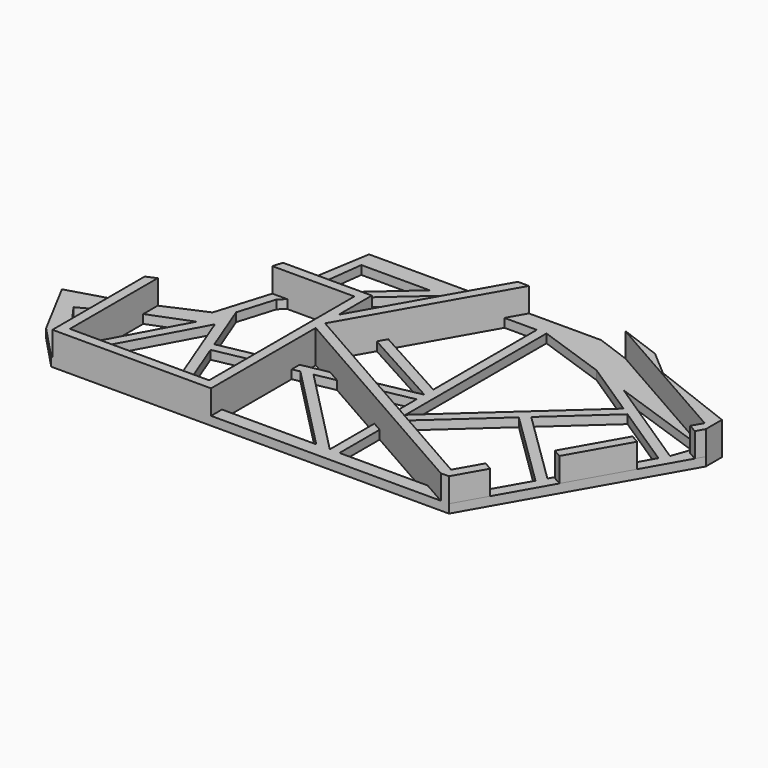
from build123d import *

# Parameters (mm, degrees)
F1_DEPTH      = 2.286
F4_DEPTH      = 2.287
F5_DEPTH      = 6.35
F5_DEPTH_BACK = 2.286


# Not quite as in the source:
# - a feature names something its author has since deleted; it is built from what else it names


with BuildPart() as f1:
    # F0 (on Top) → F1 (new body)
    with BuildSketch(Plane.XY):
        Polygon((-39.7502322496, -19.8751161248), (-31.0001806734, -29.1251689516), (73.3058652154, -29.1251689516), (101.3186621261, 20.063493978), (101.3186621261, 25.3395497125), (78.8771229202, 34.0285638846), (72.3271246897, 39.6729167182), (52.3297434038, 47.023841916), (50.4247434038, 47.023841916), (21.8864718038, 47.023841916), (19.9814718038, 47.023841916), (-8.5567997962, 47.023841916), (-12.4402794499, 23.3751358177), (-17.5001015898, 6.8750406358), (-33.2501941145, 0), (-48.0002794499, -4.3750257881), align=None)
    extrude(amount=F1_DEPTH)

    # F3 (on face) → F4 (cut, through all)
    with BuildSketch(Plane.XY.offset(2.286)):
        Polygon((-1.4134727199, 27.9240615151), (-10.8518015695, 19.606512621), (-13.772583649, 9.942060765), (-8.389721466, -3.9236969292), (39.1813585612, 5.4958437045), align=None)
        Polygon((39.1813585612, 42.3302979083), (14.9339871262, 42.3302979083), (0.6105190133, 29.707708861), (39.1813585612, 8.3977252198), align=None)
        Polygon((59.9464575784, 35.9643820735), (41.7213585612, 42.3302979083), (41.7213585612, -3.8873157464), (74.8655756118, 26.1523920247), align=None)
        Polygon((94.1682944652, 13.4573999427), (77.0573760218, 24.7108910081), (62.4269453342, 11.4508444138), (82.0611413863, -7.8019792523), align=None)
        Polygon((97.8877921519, 22.7117055132), (69.8045753566, 32.5210017107), (95.4278561797, 15.6691089989), align=None)
        Polygon((60.5416469817, 9.7421357277), (41.7213585612, -7.3153184719), (41.7213585612, -25.5348474687), (71.9623257974, -25.5348474687), (80.7611698183, -10.0846454022), align=None)
        Polygon((39.1813585612, -25.5348474687), (39.1813585612, 2.906528429), (15.8625438549, -1.7108256973), align=None)
        Polygon((12.8853386979, -2.3003415321), (-7.4562708514, -6.3281798236), (0, -25.5348474687), (35.6271387151, -25.5348474687), align=None)
        Polygon((-2.7246861202, -25.5348474687), (-13.8299450744, 3.0712777777), (-29.3522901989, -25.5348474687), align=None)
        Polygon((-31.0001806734, -23.2460485454), (-17.5001015898, 1.6332432115), (-31.0001806734, -3.6563351177), (-41.1958687779, -9.0849860736), align=None)
        Polygon((11.0922382598, 42.3302979083), (-6.8430267274, 42.3302979083), (-8.8859712705, 26.1111650616), (-9.4571967621, 24.2210612772), align=None)
    extrude(amount=-F4_DEPTH, mode=Mode.SUBTRACT)

    # F2 (on face) → F5 (join, two sides)
    with BuildSketch(Plane.XY.offset(2.286)) as f5_sk:
        Polygon((75.6003040089, -19.9636537803), (71.829370857, -26.5851689516), (11.132148453, 7.9817182735), (33.3665214857, 47.023841916), (30.4435046989, 47.023841916), (10.9098193266, 12.7239514546), (10.9098193266, 23.5798310484), (-12.3775088144, 23.5798310484), (-12.4402794499, 23.3751358177), (-13.1564102749, 21.0398310484), (8.3698193266, 21.0398310484), (8.3698193266, -26.5851689516), (-28.1426806734, -26.5851689516), (-28.1426806734, 2.2294702333), (-30.6826806734, 1.1207400345), (-30.6826806734, -29.1251689516), (-28.1426806734, -29.1251689516), (8.3698193266, -29.1251689516), (10.9098193266, -29.1251689516), (10.9098193266, 5.1853172614), (71.1568181061, -29.1251689516), (73.3058652154, -29.1251689516), (77.8074757327, -21.2206314976), align=None)
        Polygon((91.6267699042, 8.177785698), (83.1421703125, -6.7206234376), (85.3493420363, -7.9776011549), (93.8339416279, 6.9208079807), align=None)
        Polygon((99.4828806371, 21.9726089716), (97.9116584905, 19.2136443169), (100.1188302143, 17.9566665996), (101.3186621261, 20.063493978), (101.3186621261, 25.3395497125), (78.8771229202, 34.0285638846), (72.3271246897, 39.6729167182), (61.2565125507, 43.7424116468), align=None)
    extrude(amount=F5_DEPTH)
    extrude(f5_sk.sketch, amount=-F5_DEPTH_BACK)


solid = f1.part
